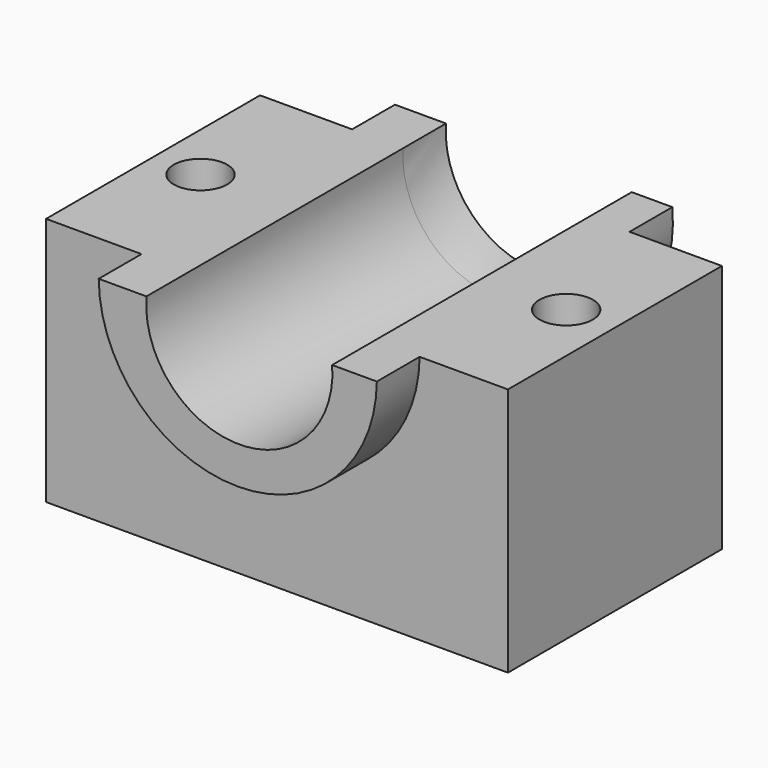
from build123d import *
from build123d import SkipClean  # not in build123d's __all__

# Parameters (mm, degrees)
F1_DEPTH = 63.5
F3_DEPTH = 12.7
F4_DEPTH = 63.501
F6_DEPTH = 12.7
F8_D     = 12.7
F8_DEPTH = 152.4
F8_TIP   = 3.8154649308


# Not quite as in the source:
# - after a boolean that leaves OpenCascade's solid faulty, fix() repairs it


with BuildPart() as f1:
    # F0 (on Front) → F1 (new body)
    with BuildSketch(Plane.XZ):
        Polygon((-29.9473897851, 37.1472596026), (-42.7499328044, 37.1472596026), (-55.5491112173, 37.1472596026), (-55.5491112173, -22.0509488136), (54.1031509638, -22.0509488136), (54.1031509638, 37.1472596026), (41.2416318434, 37.1472596026), (28.4390888242, 37.1472596026), (20.3639920801, 37.1472596026), (-23.0149235576, 37.1472596026), align=None)
    extrude(amount=-F1_DEPTH)

    # F2 (on face) → F3 (join)
    with BuildSketch(Plane.XZ):
        with BuildLine():
            Line((-21.5689614415, 37.1472596026), (-32.8956767917, 37.1472596026))
            ThreePointArc((-32.8956767917, 37.1472596026), (0.1204963773, 4.4575092605), (33.1366695464, 37.1472596026))
            Line((33.1366695464, 37.1472596026), (22.5329399109, 37.1472596026))
            ThreePointArc((22.5329399109, 37.1472596026), (0.4819892347, 13.3748375843), (-21.5689614415, 37.1472596026))
        make_face()
    extrude(amount=F3_DEPTH)

    # F4 (cut, through all): a face of the model
    f4_faces = [f1.faces().sort_by_distance(p)[0] for p in [
        (0.4819892347, 0, 26.9928771395),
    ]]
    extrude(f4_faces, amount=-F4_DEPTH, mode=Mode.SUBTRACT)

    # F5 (on face) → F6 (join)
    with BuildSketch(Plane(origin=(0, 63.5, 0), x_dir=(-1, 0, 0), z_dir=(0, 1, 0))):
        with BuildLine():
            Line((-22.5329399109, 37.1472596026), (-32.1724079549, 37.1472596026))
            ThreePointArc((-32.1724079549, 37.1472596026), (0.7585827261, 1.0699512778), (33.6895734072, 37.1472596026))
            Line((33.6895734072, 37.1472596026), (21.5689614415, 37.1472596026))
            ThreePointArc((21.5689614415, 37.1472596026), (-0.4819892347, 13.3748375843), (-22.5329399109, 37.1472596026))
        make_face()
    with SkipClean():  # cleaning this boolean's faces spoils the solid; the shape is the same uncleaned
        extrude(amount=F6_DEPTH)

    # F8
    with Locations(Plane.XY.offset(37.1472596026)):
        with Locations((-44.2922338843, 31.75), (42.5287522376, 31.75)):
            Hole(F8_D / 2, depth=F8_DEPTH)
            with Locations((0, 0, -(F8_DEPTH + F8_TIP / 2))):  # 118° drill point
                Cone(0, F8_D / 2, F8_TIP, mode=Mode.SUBTRACT)

    add(f1.part.fix(), mode=Mode.REPLACE)


solid = f1.part
